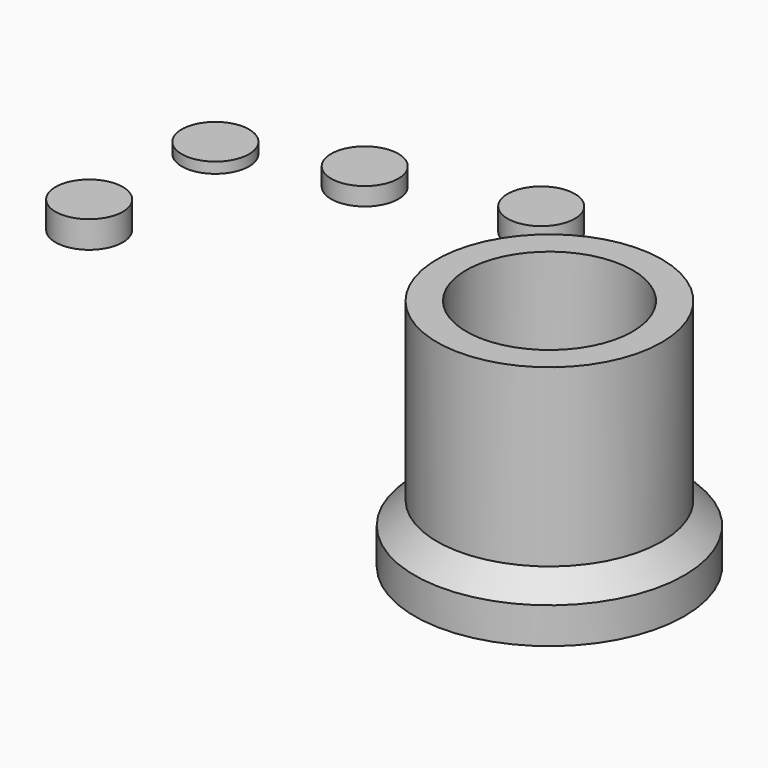
from build123d import *

# Parameters (mm, degrees)
F0_R      = 3.74
F1_DEPTH  = 1.2
F2_R      = 3.74
F3_DEPTH  = 2
F4_R      = 3.74
F5_DEPTH  = 2.5
F6_R      = 3.74
F7_DEPTH  = 3
F8_R      = 15
F8_R_2    = 9.25
F9_DEPTH  = 26
F10_R     = 15
F10_R_2   = 12.5
F11_DEPTH = 22
F12_SIZE  = 2.49999


# Not quite as in the source:
# - a fillet or chamfer is up to 0.001 mm smaller than in the source, because OpenCascade refuses the exact size


with BuildPart() as f1:
    # F0 (on Top) → F1 (new body)
    with BuildSketch(Plane.XY):
        with Locations((-71.0977017879, 42.4381643534)):
            Circle(F0_R)
    extrude(amount=F1_DEPTH)


with BuildPart() as f3:
    # F2 (on Top) → F3 (new body)
    with BuildSketch(Plane.XY):
        with Locations((-57.1353621781, 45.7450337708)):
            Circle(F2_R)
    extrude(amount=F3_DEPTH)


with BuildPart() as f5:
    # F4 (on Top) → F5 (new body)
    with BuildSketch(Plane.XY):
        with Locations((-39.8661494255, 48.6844740808)):
            Circle(F4_R)
    extrude(amount=F5_DEPTH)


with BuildPart() as f7:
    # F6 (on Top) → F7 (new body)
    with BuildSketch(Plane.XY):
        with Locations((-70.7302689552, 24.4340933859)):
            Circle(F6_R)
    extrude(amount=F7_DEPTH)


with BuildPart() as f9:
    # F8 (on Top) → F9 (new body)
    with BuildSketch(Plane.XY):
        Circle(F8_R)
        Circle(F8_R_2, mode=Mode.SUBTRACT)
    extrude(amount=F9_DEPTH)

    # F10 (on face) → F11 (cut)
    with BuildSketch(Plane.XY.offset(26)):
        Circle(F10_R)
        Circle(F10_R_2, mode=Mode.SUBTRACT)
    extrude(amount=-F11_DEPTH, mode=Mode.SUBTRACT)

    # F12 (size 2.5 in the source; OpenCascade refuses exactly that, so slightly less here)
    f12_edges = [f9.edges().sort_by_distance(p)[0] for p in [
        (-12.5, 0, 4),
    ]]
    chamfer(f12_edges, length=F12_SIZE)


solid = Compound([f1.part, f3.part, f5.part, f7.part, f9.part])
